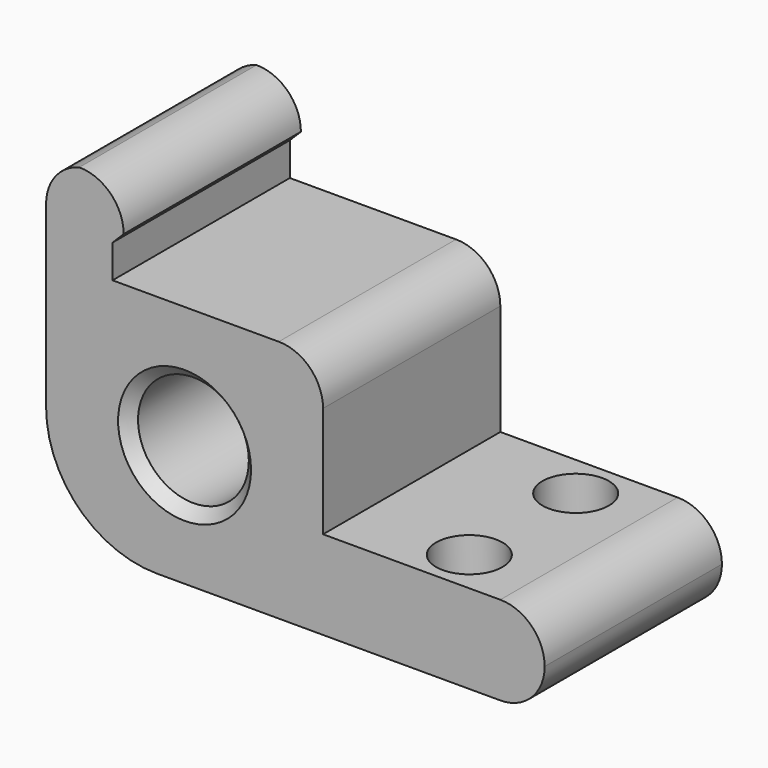
from build123d import *

# Parameters (mm, degrees)
F0_R        = 2.5
F1_DEPTH    = 10
F2_R        = 1.5
F3_DEPTH    = 25
F4_R        = 1.99999
F5_T1_DEPTH = 19.6824712753
F6_R        = 5
F7_R        = 2
F8_R        = 1.99999
F9_SIZE     = 0.49999
F10_SIZE    = 0.5


# Not quite as in the source:
# - a fillet or chamfer that OpenCascade refuses, or shapes differently, is made with other operations: its cross-section is extruded or revolved along the edge and cut away or added
# - a fillet or chamfer is up to 0.001 mm smaller than in the source, because OpenCascade refuses the exact size


with BuildPart() as f1:
    # F0 (on Front) → F1 (new body)
    with BuildSketch(Plane.XZ):
        Polygon((-2.75, 9.5), (-6.25, 9.5), (-6.25, -5.5), (16.25, -5.5), (16.25, -1.5), (6.25, -1.5), (6.25, 5.5), (-3.25, 5.5), (-3.25, 7), (-2.75, 7.5), align=None)
        Circle(F0_R, mode=Mode.SUBTRACT)
    extrude(amount=F1_DEPTH)

    # F2 (on face) → F3 (cut)
    with BuildSketch(Plane.XY.offset(-1.5)):
        with Locations((11.25, -8)):
            Circle(F2_R)
        with Locations((11.25, -2)):
            Circle(F2_R)
    extrude(amount=-F3_DEPTH, mode=Mode.SUBTRACT)

    # F4 (radius 2 in the source; OpenCascade refuses exactly that, so slightly less here)
    f4_edges = [f1.edges().sort_by_distance(p)[0] for p in [
        (-2.75, -5, 9.5),
    ]]
    fillet(f4_edges, radius=F4_R)

    # F5: fillet of radius 2 on 1 edges, made by hand

    # F5_s2 → F5_t1 (cut)
    with BuildSketch(Plane.XZ.offset(-4.8412356377)):
        with BuildLine():
            ThreePointArc((-4.74999, 9.5), (-5.8311356678, 8.7882546988), (-6.25, 7.5635057449))
            Line((-6.25, 7.5635057449), (-6.25, 9.5))
            Line((-6.25, 9.5), (-4.74999, 9.5))
        make_face()
    extrude(amount=F5_T1_DEPTH, mode=Mode.SUBTRACT)

    # F6
    f6_edges = [f1.edges().sort_by_distance(p)[0] for p in [
        (-6.25, -5, -5.5),
    ]]
    fillet(f6_edges, radius=F6_R)

    # F7
    f7_edges = [f1.edges().sort_by_distance(p)[0] for p in [
        (6.25, -5, 5.5),
    ]]
    fillet(f7_edges, radius=F7_R)

    # F8 (radius 2 in the source; OpenCascade refuses exactly that, so slightly less here)
    f8_edges = [f1.edges().sort_by_distance(p)[0] for p in [
        (16.25, -5, -1.5),
        (16.25, -5, -5.5),
    ]]
    fillet(f8_edges, radius=F8_R)

    # F9 (size 0.5 in the source; OpenCascade refuses exactly that, so slightly less here)
    f9_edges = [f1.edges().sort_by_distance(p)[0] for p in [
        (9.75, -8, -5.5),
        (9.75, -2, -5.5),
    ]]
    chamfer(f9_edges, length=F9_SIZE)

    # F10
    f10_edges = [f1.edges().sort_by_distance(p)[0] for p in [
        (-2.5, -10, 0),
        (-2.5, 0, 0),
    ]]
    chamfer(f10_edges, length=F10_SIZE)


solid = f1.part
